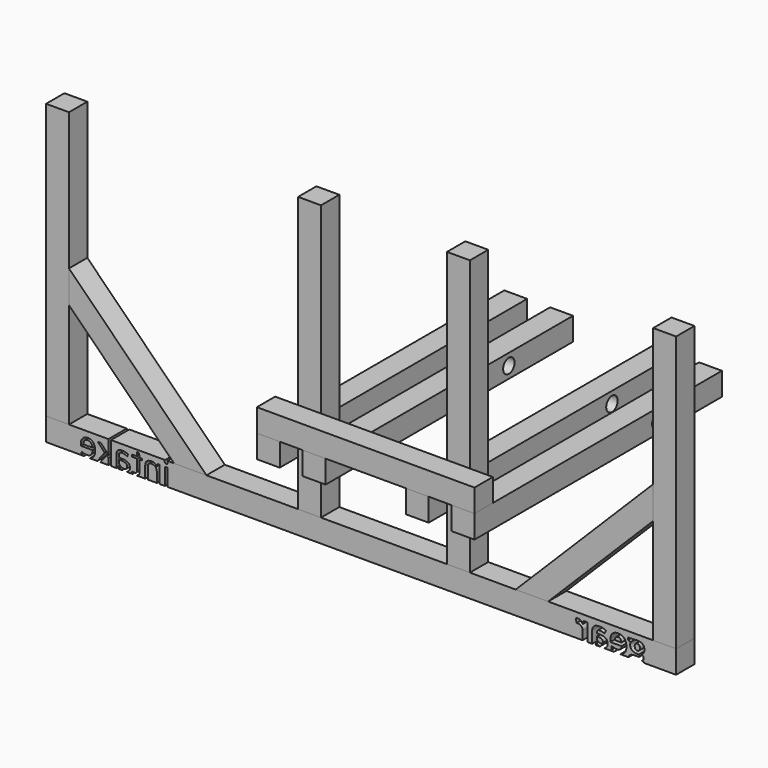
from build123d import *

# Parameters (mm, degrees)
F3_W           = 25.4
F3_H           = 25.4
F4_DEPTH       = 304.8
F5_W           = 698.5
F5_H           = 25.4
F6_DEPTH       = 12.7
F7_TEXT_SIZE   = 35.2777777778
F8_DEPTH       = 25.401
F10_DEPTH      = 12.7
F11_W          = 25.4
F11_H          = 25.4
F12_DEPTH      = 38.1
F12_DEPTH_BACK = 304.8
F13_W          = 241.3
F13_H          = 25.4
F14_DEPTH      = 25.4
F15_R          = 7.9375
F16_DEPTH      = 495.3010001


# Not quite as in the source:
# - Text() gives the source's letters only with a copy of the font that has no kerning and outlines rounded to 1/6400 em; it was checked with that copy


with BuildPart() as f4:
    # F3 (on Top) → F4 (new body)
    with BuildSketch(Plane.XY):
        with Locations((-336.55, 0)):
            Rectangle(F3_W, F3_H)
    extrude(amount=F4_DEPTH)


with BuildPart() as f4b:
    # F3 (on Top) → F4, piece 2 (new body)
    with BuildSketch(Plane.XY):
        with Locations((-57.15, 0)):
            Rectangle(F3_W, F3_H)
    extrude(amount=F4_DEPTH)


with BuildPart() as f4c:
    # F3 (on Top) → F4, piece 3 (new body)
    with BuildSketch(Plane.XY):
        with Locations((107.95, 0)):
            Rectangle(F3_W, F3_H)
    extrude(amount=F4_DEPTH)


with BuildPart() as f4d:
    # F3 (on Top) → F4, piece 4 (new body)
    with BuildSketch(Plane.XY):
        with Locations((336.55, 0)):
            Rectangle(F3_W, F3_H)
    extrude(amount=F4_DEPTH)


with BuildPart() as f6:
    # F5 (on Front) → F6 (new body, symmetric)
    with BuildSketch(Plane.XZ):
        with Locations((0, -12.7)):
            Rectangle(F5_W, F5_H)
    extrude(amount=F6_DEPTH, both=True)

    # F7 (on face) → F8 (cut, through all)
    with BuildSketch(Plane(origin=(0, 12.7, 0), x_dir=(-1, 0, 0), z_dir=(0, 1, 0))):
        with Locations((-315.6553208828, -25.4)):
            Text('gear', F7_TEXT_SIZE, font='Open Sans', font_style=FontStyle.BOLD, text_align=(TextAlign.LEFT, TextAlign.BOTTOM))
        with Locations((211.6142958403, -25.4)):
            Text('intake', F7_TEXT_SIZE, font='Open Sans', text_align=(TextAlign.LEFT, TextAlign.BOTTOM))
    extrude(amount=-F8_DEPTH, mode=Mode.SUBTRACT)


with BuildPart() as f10:
    # F9 (on Front) → F10 (new body, symmetric)
    with BuildSketch(Plane.XZ):
        Polygon((323.85, 152.4), (171.45, 0), (207.3710244843, 0), (323.85, 116.4789755157), align=None)
    extrude(amount=F10_DEPTH, both=True)


with BuildPart() as f10b:
    # F9 (on Front) → F10, piece 2 (new body, symmetric)
    with BuildSketch(Plane.XZ):
        Polygon((-207.3710244843, 0), (-171.45, 0), (-323.85, 152.4), (-323.85, 116.4789755157), align=None)
    extrude(amount=F10_DEPTH, both=True)


with BuildPart() as f12:
    # F11 (on Front) → F12 (new body, two sides)
    with BuildSketch(Plane.XZ) as f12_sk:
        with Locations((133.35, 63.5)):
            Rectangle(F11_W, F11_H)
    extrude(amount=F12_DEPTH)
    extrude(f12_sk.sketch, amount=-F12_DEPTH_BACK)


with BuildPart() as f12b:
    # F11 (on Front) → F12, piece 2 (new body, two sides)
    with BuildSketch(Plane.XZ) as f12_2_sk:
        with Locations((82.55, 63.5)):
            Rectangle(F11_W, F11_H)
    extrude(amount=F12_DEPTH)
    extrude(f12_2_sk.sketch, amount=-F12_DEPTH_BACK)


with BuildPart() as f12c:
    # F11 (on Front) → F12, piece 3 (new body, two sides)
    with BuildSketch(Plane.XZ) as f12_3_sk:
        with Locations((-31.75, 63.5)):
            Rectangle(F11_W, F11_H)
    extrude(amount=F12_DEPTH)
    extrude(f12_3_sk.sketch, amount=-F12_DEPTH_BACK)


with BuildPart() as f12d:
    # F11 (on Front) → F12, piece 4 (new body, two sides)
    with BuildSketch(Plane.XZ) as f12_4_sk:
        with Locations((-82.55, 63.5)):
            Rectangle(F11_W, F11_H)
    extrude(amount=F12_DEPTH)
    extrude(f12_4_sk.sketch, amount=-F12_DEPTH_BACK)


with BuildPart() as f14:
    # F13 (on face) → F14 (new body)
    with BuildSketch(Plane.XY.offset(76.2)):
        with Locations((25.4, -25.4)):
            Rectangle(F13_W, F13_H)
    extrude(amount=F14_DEPTH)


with BuildPart() as f16_tool:
    # F15 (on face) → F16 (new body, through all)
    with BuildSketch(Plane.YZ.offset(146.05)):
        with Locations((215.9, 63.5)):
            Circle(F15_R)
    extrude(amount=-F16_DEPTH)


with BuildPart() as f12_1:
    add(f12.part)

    # F16: cut by f16_tool
    add(f16_tool.part, mode=Mode.SUBTRACT)


with BuildPart() as f12b_1:
    add(f12b.part)

    # F16: cut by f16_tool
    add(f16_tool.part, mode=Mode.SUBTRACT)


with BuildPart() as f12c_1:
    add(f12c.part)

    # F16: cut by f16_tool
    add(f16_tool.part, mode=Mode.SUBTRACT)


with BuildPart() as f12d_1:
    add(f12d.part)

    # F16: cut by f16_tool
    add(f16_tool.part, mode=Mode.SUBTRACT)


solid = Compound([f4.part, f4b.part, f4c.part, f4d.part, f6.part, f10.part, f10b.part, f14.part, f12_1.part, f12b_1.part, f12c_1.part, f12d_1.part])
